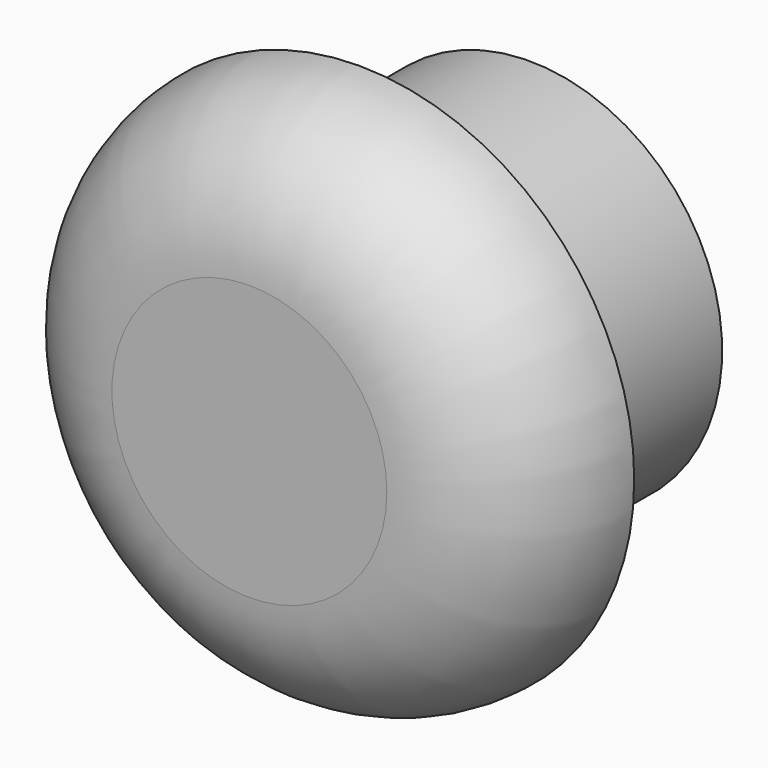
from build123d import *

# Parameters (mm, degrees)
F0_R     = 4
F1_DEPTH = 2
F2_R     = 1.99999
F3_R     = 2.8
F4_DEPTH = 3.1
F5_R     = 1.5
F6_DEPTH = 3


# Not quite as in the source:
# - a fillet or chamfer is up to 0.001 mm smaller than in the source, because OpenCascade refuses the exact size


with BuildPart() as f1:
    # F0 (on Front) → F1 (new body)
    with BuildSketch(Plane.XZ):
        Circle(F0_R)
    extrude(amount=F1_DEPTH)

    # F2 (radius 2 in the source; OpenCascade refuses exactly that, so slightly less here)
    f2_edges = [f1.edges().sort_by_distance(p)[0] for p in [
        (-4, -2, 0),
    ]]
    fillet(f2_edges, radius=F2_R)

    # F3 (on face) → F4 (join)
    with BuildSketch(Plane(origin=(0, 0, 0), x_dir=(-1, 0, 0), z_dir=(0, 1, 0))):
        Circle(F3_R)
    extrude(amount=F4_DEPTH)

    # F5 (on face) → F6 (cut)
    with BuildSketch(Plane(origin=(0, 3.1, 0), x_dir=(-1, 0, 0), z_dir=(0, 1, 0))):
        with Locations((0.0365495689, 0.0300457796)):
            Circle(F5_R)
    extrude(amount=-F6_DEPTH, mode=Mode.SUBTRACT)


solid = f1.part
